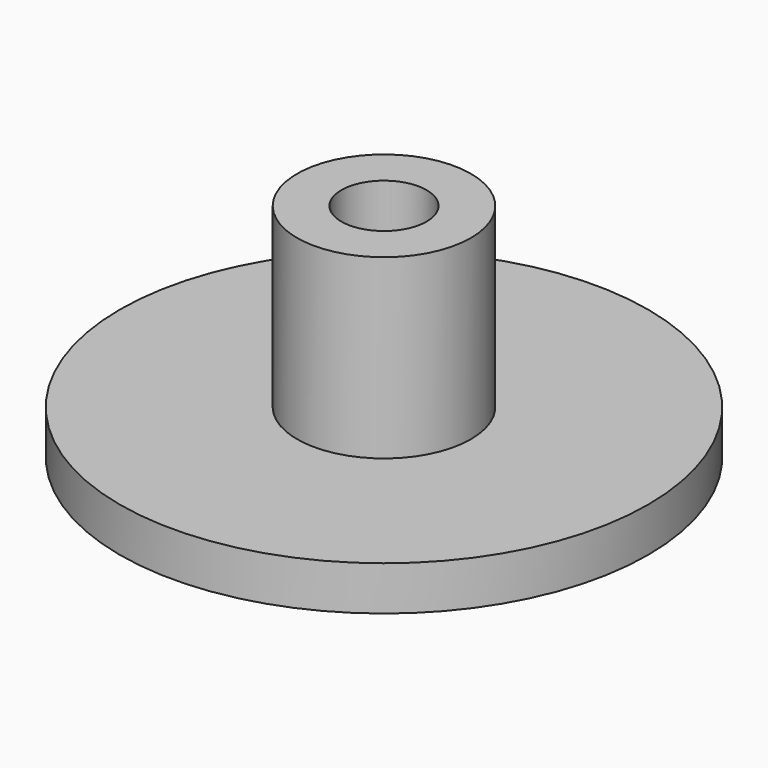
from build123d import *


# Not quite as in the source:
# - ends of sketch curves that miss each other by under 0.0002 mm in the source are joined


with BuildPart() as f1:
    # F0 (on Front) → F1 (revolve)
    with BuildSketch(Plane.XZ):
        Polygon((9.6277087807, 50.3076042631), (9.6277087807, 0.3076042631), (59.6277085234, 0.3126767645), (59.6277085234, 10.3076042631), (19.6277087807, 10.3076042631), (19.6277087807, 50.3076042631), align=None)
    revolve(axis=Axis((0, 0, 31.0427118093), (0, 0, 1)))


solid = f1.part
